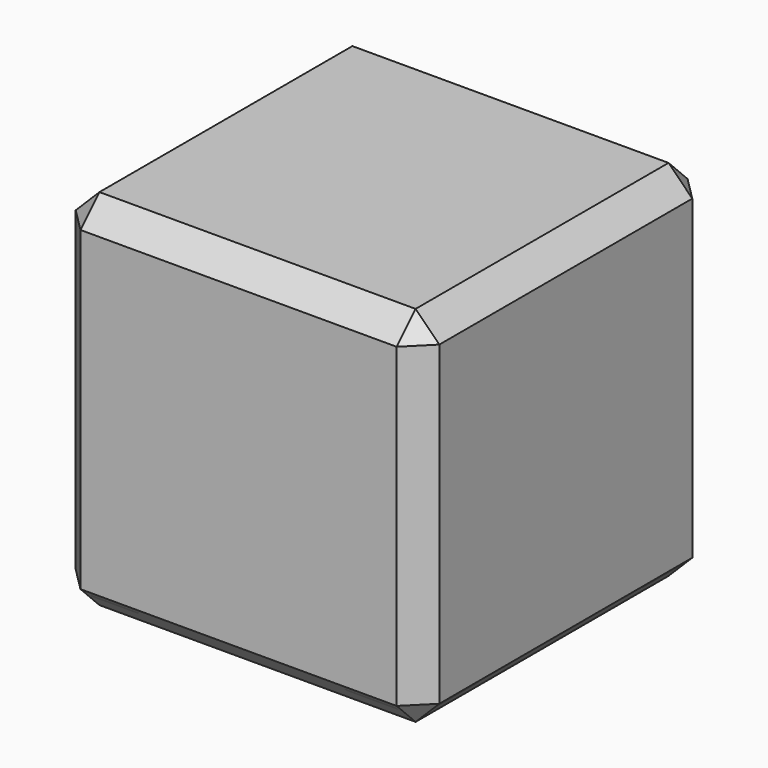
from build123d import *

# Parameters (mm, degrees)
F0_W      = 92
F0_H      = 92
F1_DEPTH  = 92
F2_SIZE   = 6
F3_DEPTH  = 80
F4_W      = 89
F4_H      = 89
F5_DEPTH  = 89
F6_SIZE   = 6
F17_DEPTH = 3.5
F10_R     = 1.65
F11_DEPTH = 1.3
F12_SIZE  = 0.49999
F15_DEPTH = 1.5


# Not quite as in the source:
# - a fillet or chamfer is up to 0.001 mm smaller than in the source, because OpenCascade refuses the exact size


with BuildPart() as f1:
    # F0 (on Top) → F1 (new body)
    with BuildSketch(Plane.XY):
        Rectangle(F0_W, F0_H)
    extrude(amount=F1_DEPTH)

    # F2
    f2_edges = [f1.edges().sort_by_distance(p)[0] for p in [
        (0, -46, 92),
        (46, 0, 92),
        (46, -46, 46),
        (0, -46, 0),
        (-46, -46, 46),
        (46, 0, 0),
        (46, 46, 46),
        (0, 46, 92),
        (-46, 0, 92),
        (-46, 0, 0),
        (-46, 46, 46),
        (0, 46, 0),
    ]]
    chamfer(f2_edges, length=F2_SIZE)

    # F3 (cut): a face of the model
    f3_faces = [f1.faces().sort_by_distance(p)[0] for p in [
        (0, 0, 0),
    ]]
    extrude(f3_faces, amount=-F3_DEPTH, mode=Mode.SUBTRACT)


with BuildPart() as f5:
    # F4 (on Top) → F5 (new body)
    with BuildSketch(Plane.XY):
        Rectangle(F4_W, F4_H)
    extrude(amount=F5_DEPTH)

    # F6
    f6_edges = [f5.edges().sort_by_distance(p)[0] for p in [
        (-44.5, -44.5, 44.5),
        (0, -44.5, 89),
        (44.5, -44.5, 44.5),
        (0, -44.5, 0),
        (44.5, 0, 89),
        (44.5, 44.5, 44.5),
        (44.5, 0, 0),
        (0, 44.5, 0),
        (-44.5, 0, 89),
        (0, 44.5, 89),
        (-44.5, 44.5, 44.5),
        (-44.5, 0, 0),
    ]]
    chamfer(f6_edges, length=F6_SIZE)


with BuildPart() as f5_1:
    # F7: moved
    add(f5.part.moved(Location((0, 0, 1.5))))


with BuildPart() as f1_1:
    add(f1.part)

    # F8: cut F5
    add(f5_1.part, mode=Mode.SUBTRACT)

    # F16 (on offset) → F17 (join)
    with BuildSketch(Plane.XY.offset(7.5)):
        Polygon((44.5, 26.0656665673), (44.5, 38.5), (38.5, 44.5), (26.0656665673, 44.5), (30.5656665673, 40), (40.5656665673, 30), align=None)
        Polygon((-25.5, 44.5), (-38.5, 44.5), (-44.5, 38.5), (-44.5, 25.5), (-40, 30), (-30, 40), align=None)
        Polygon((25.5, -44.5), (38.5, -44.5), (44.5, -38.5), (44.5, -25.5), (40, -30), (30, -40), align=None)
        Polygon((-44.5, -38.5), (-38.5, -44.5), (-26.5405371355, -44.5), (-30, -41.0405371355), (-40, -31.0405371355), (-44.5, -26.5405371355), align=None)
    extrude(amount=-F17_DEPTH)

    # F10 (on face) → F11 (cut)
    with BuildSketch(Plane(origin=(0, 0, 4), x_dir=(1, 0, 0), z_dir=(0, 0, -1))):
        with Locations((37.4, 37.4)):
            Circle(F10_R)
        with Locations((-37.4, 37.4)):
            Circle(F10_R)
        with Locations((-37.4, -37.4)):
            Circle(F10_R)
        with Locations((37.4, -37.4)):
            Circle(F10_R)
    extrude(amount=-F11_DEPTH, mode=Mode.SUBTRACT)

    # F12 (size 0.5 in the source; OpenCascade refuses exactly that, so slightly less here)
    f12_edges = [f1_1.edges().sort_by_distance(p)[0] for p in [
        (-32, 44.5, 4),
        (-44.5, 32, 4),
        (32.282833, 44.5, 4),
        (44.5, 32.282833, 4),
        (44.5, -32, 4),
        (-32.520269, -44.5, 4),
        (-44.5, -32.520269, 4),
        (32, -44.5, 4),
    ]]
    chamfer(f12_edges, length=F12_SIZE)

    # F14 (on face) → F15 (join)
    with BuildSketch(Plane(origin=(0, 0, 3), x_dir=(1, 0, 0), z_dir=(0, 0, -1))):
        Polygon((-41, 38.5), (-41, 30.0405371355), (-40, 31.0405371355), (-40, 39.5), (-40, 40), (-39.5, 40), (-31.0405371355, 40), (-30.0405371355, 41), (-38.5, 41), (-40, 41), (-41, 40), align=None)
        Polygon((38.5, 41), (29, 41), (30, 40), (39.5, 40), (40, 40), (40, 39.5), (40, 30), (41, 29), (41, 38.5), (41, 40), (40, 41), align=None)
        Polygon((41, -38.5), (41, -29.5656665673), (40, -30.5656665673), (40, -40), (30.5656665673, -40), (29.5656665673, -41), (38.5, -41), (40, -41), (41, -40), align=None)
        Polygon((-38.5, -41), (-29, -41), (-30, -40), (-40, -40), (-40, -30), (-41, -29), (-41, -38.5), (-41, -40), (-40, -41), align=None)
    extrude(amount=-F15_DEPTH)


solid = f1_1.part
